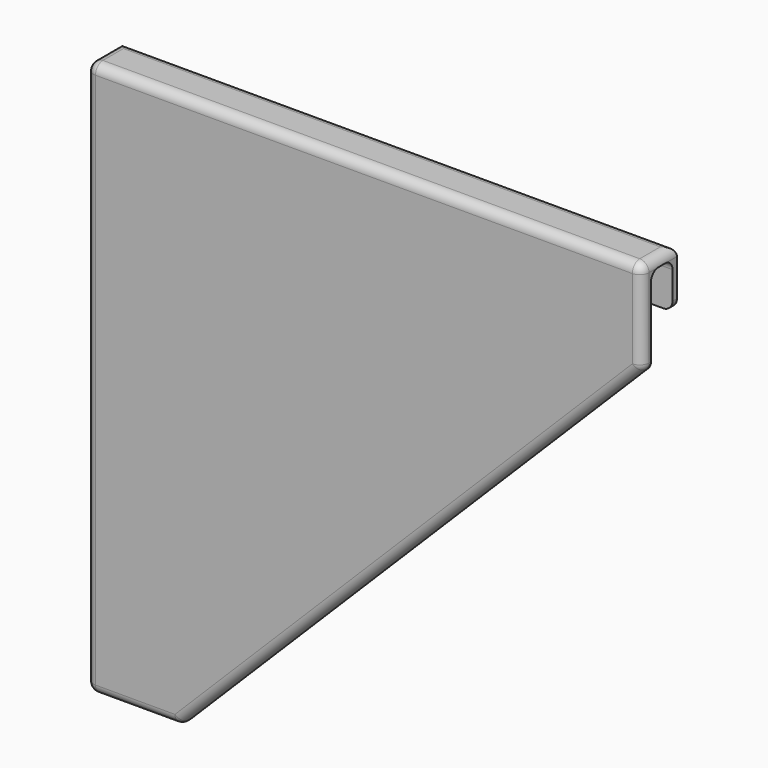
from build123d import *

# Parameters (mm, degrees)
F1_W     = 120
F1_H     = 2
F2_DEPTH = 7
F3_DEPTH = 2.54
F4_W     = 120
F4_H     = 1.2
F5_DEPTH = 10
F6_R     = 1.9999


# Not quite as in the source:
# - a fillet or chamfer is up to 0.001 mm smaller than in the source, because OpenCascade refuses the exact size


with BuildPart() as f2:
    # F1 (on face) → F2 (new body)
    with BuildSketch(Plane.XZ):
        with Locations((60, 119)):
            Rectangle(F1_W, F1_H)
    extrude(amount=-F2_DEPTH)

    # F0 (on Front) → F3 (join)
    with BuildSketch(Plane.XZ):
        Polygon((0, 120), (0, 0), (20, 0), (120, 100), (120, 120), align=None)
    extrude(amount=F3_DEPTH)

    # F4 (on face) → F5 (join)
    with BuildSketch(Plane(origin=(0, 0, 118), x_dir=(1, 0, 0), z_dir=(0, 0, -1))):
        with Locations((60, -6.4)):
            Rectangle(F4_W, F4_H)
    extrude(amount=F5_DEPTH)

    # F6 (radius 2 in the source; OpenCascade refuses exactly that, so slightly less here)
    f6_edges = [f2.edges().sort_by_distance(p)[0] for p in [
        (0, -1.27, 0),
        (20, -1.27, 0),
        (120, -1.27, 100),
        (0, 2.23, 120),
        (120, 2.23, 120),
        (120, 6.4, 108),
        (0, 6.4, 108),
        (0, -2.54, 60),
        (60, -2.54, 120),
        (120, -2.54, 110),
        (70, -2.54, 50),
        (10, -2.54, 0),
        (60, 0, 118),
        (60, 5.8, 118),
        (60, 7, 120),
    ]]
    fillet(f6_edges, radius=F6_R)


solid = f2.part
